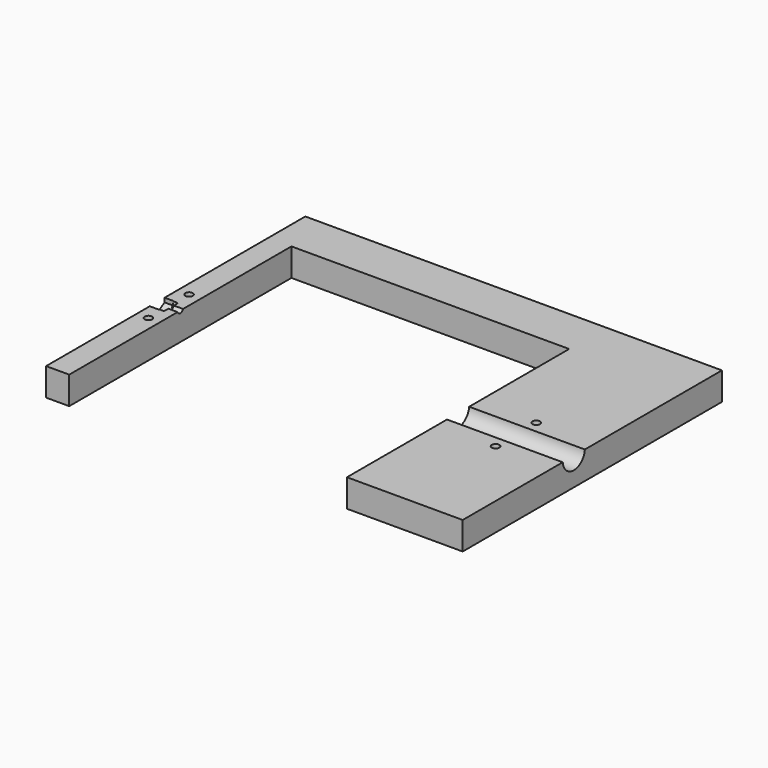
from build123d import *

# Parameters (mm, degrees)
F0_W      = 180
F0_H      = 140
F1_DEPTH  = 30
F4_DEPTH  = 30
F5_DEPTH  = 4
F6_R      = 3.8
F7_DEPTH  = 2
F8_R      = 1.55
F9_DEPTH  = 7
F10_R     = 6
F12_DEPTH = 50
F11_R     = 0.5
F13_DEPTH = 1
F14_W     = 180
F14_H     = 140
F15_DEPTH = 18
F16_R     = 1.65
F17_DEPTH = 12


# Not quite as in the source:
# - a feature names something its author has since deleted; it is built from what else it names


with BuildPart() as f1:
    # F0 (on Top) → F1 (new body)
    with BuildSketch(Plane.XY):
        Rectangle(F0_W, F0_H)
    extrude(amount=F1_DEPTH)

    # F3 (on Top) → F4 (cut, through all)
    with BuildSketch(Plane.XY):
        Polygon((40, -70), (40, 0), (40, 50), (0, 50), (-80, 50), (-80, -70), align=None)
    extrude(amount=F4_DEPTH, mode=Mode.SUBTRACT)

    # F2 (on face) → F5 (cut)
    with BuildSketch(Plane(origin=(-90, 0, 0), x_dir=(0, -1, 0), z_dir=(-1, 0, 0))):
        Polygon((10, 17.12), (5.9989626345, 14.81), (5.9989626345, 10.19), (10, 7.88), (14.0010373655, 10.19), (14.0010373655, 14.81), align=None)
    extrude(amount=-F5_DEPTH, mode=Mode.SUBTRACT)

    # F6 (on face) → F7 (cut)
    with BuildSketch(Plane(origin=(-86, 0, 0), x_dir=(0, -1, 0), z_dir=(-1, 0, 0))):
        with Locations((10, 12.5)):
            Circle(F6_R)
    extrude(amount=-F7_DEPTH, mode=Mode.SUBTRACT)

    # F8 (on face) → F9 (cut)
    with BuildSketch(Plane(origin=(-84, 0, 0), x_dir=(0, -1, 0), z_dir=(-1, 0, 0))):
        with Locations((10, 12.5)):
            Circle(F8_R)
    extrude(amount=-F9_DEPTH, mode=Mode.SUBTRACT)

    # F10 (on face) → F12 (cut, through all)
    with BuildSketch(Plane.YZ.offset(90)):
        with Locations((-10, 12.5)):
            Circle(F10_R)
    extrude(amount=-F12_DEPTH, mode=Mode.SUBTRACT)

    # F11 (on face) → F13 (cut)
    with BuildSketch(Plane(origin=(0, 70, 0), x_dir=(-1, 0, 0), z_dir=(0, 1, 0))):
        with Locations((35, 6)):
            Circle(F11_R)
        with Locations((10, 6)):
            Circle(F11_R)
    extrude(amount=-F13_DEPTH, mode=Mode.SUBTRACT)

    # F14 (on face) → F15 (cut)
    with BuildSketch(Plane.XY.offset(30)):
        Rectangle(F14_W, F14_H)
    extrude(amount=-F15_DEPTH, mode=Mode.SUBTRACT)

    # F16 (on face) → F17 (cut, through all)
    with BuildSketch(Plane.XY.offset(12)):
        with Locations((65, 1)):
            Circle(F16_R)
        with Locations((65, -21)):
            Circle(F16_R)
        with Locations((-85, 1)):
            Circle(F16_R)
        with Locations((-85, -21)):
            Circle(F16_R)
    extrude(amount=-F17_DEPTH, mode=Mode.SUBTRACT)


solid = f1.part
